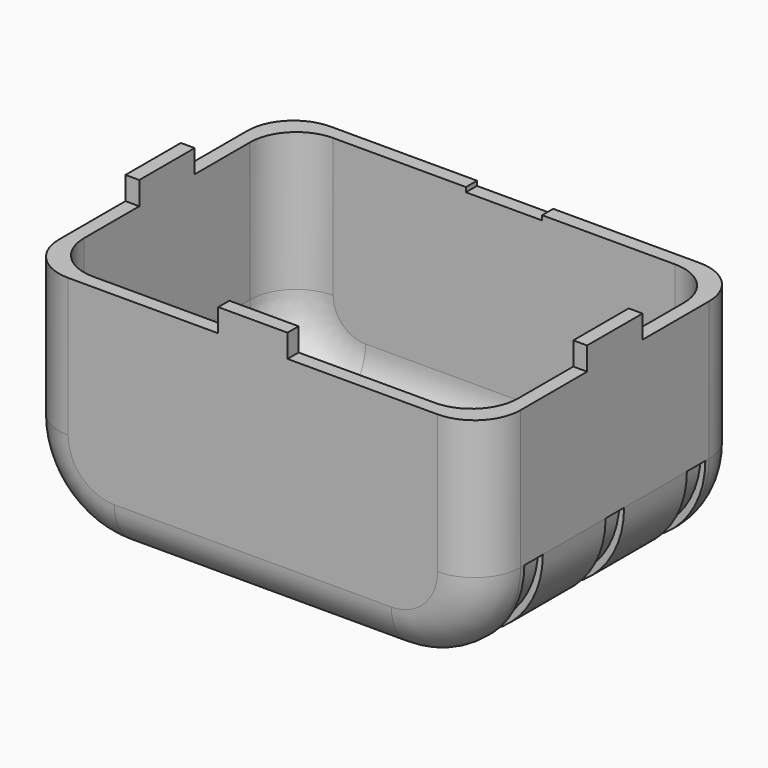
from build123d import *

# Parameters (mm, degrees)
F0_W          = 100
F0_H          = 71
F0_W_2        = 85
F0_H_2        = 56
F1_DEPTH      = 55
F2_R          = 20
F3_T          = -3
F5_DEPTH      = 60
F6_DEPTH      = 55
F7_DEPTH      = 38
F8_DEPTH      = 33
F9_DEPTH      = 16
F10_DEPTH     = 11
F11_W         = 5
F11_H         = 5
F11_W_2       = 7.5
F11_W_3       = 30
F11_W_4       = 5.0000003725
F11_W_5       = 4.9999996275
F11_H_2       = 3
F11_W_6       = 2.5
F12_DEPTH     = 1
F13_R         = 15
F14_DEPTH     = 0.5
F15_W         = 15
F15_H         = 3
F16_DEPTH     = 5
F17_W         = 16.5
F17_H         = 3
F18_DEPTH     = 1
F19_T1_DEPTH  = 60
F19_T3_DEPTH  = 30
F19_T6_ANGLE  = 90
F19_T8_ANGLE  = 90
F19_T10_ANGLE = 90
F19_T12_ANGLE = 90
F19_T13_DEPTH = 60
F19_T15_DEPTH = 55
F19_T18_ANGLE = 90
F19_T20_ANGLE = 90
F19_T22_ANGLE = 90
F19_T24_ANGLE = 90


# Not quite as in the source:
# - a fillet or chamfer that OpenCascade refuses, or shapes differently, is made with other operations: its cross-section is extruded or revolved along the edge and cut away or added
# - ends of sketch curves that miss each other by under 0.0002 mm in the source are joined


with BuildPart() as f1:
    # F0 (on Top) → F1 (new body)
    with BuildSketch(Plane.XY):
        Rectangle(F0_W, F0_H)
        Rectangle(F0_W_2, F0_H_2, mode=Mode.SUBTRACT)
        Rectangle(F0_W_2, F0_H_2)
    extrude(amount=F1_DEPTH)

    # F2
    f2_edges = [f1.edges().sort_by_distance(p)[0] for p in [
        (-50, 0, 0),
        (50, 0, 0),
    ]]
    fillet(f2_edges, radius=F2_R)

    # F3
    f3_openings = [f1.faces().sort_by_distance(p)[0] for p in [
        (0, 0, 55),
    ]]
    offset(amount=F3_T, openings=f3_openings)

    # F4 (on face) → F5 (cut)
    with BuildSketch(Plane(origin=(0, 35.5, 0), x_dir=(-1, 0, 0), z_dir=(0, 1, 0))):
        with BuildLine():
            Line((-49, 21), (-50, 20))
            ThreePointArc((-50, 20), (-44.1421356237, 5.8578643763), (-30, 0))
            Line((-30, 0), (-29, 1))
            ThreePointArc((-29, 1), (-43.1421356237, 6.8578643763), (-49, 21))
        make_face()
        with BuildLine():
            ThreePointArc((30, 0), (44.1421356237, 5.8578643763), (50, 20))
            Line((50, 20), (49, 21))
            ThreePointArc((49, 21), (43.1421356237, 6.8578643763), (29, 1))
            Line((29, 1), (30, 0))
        make_face()
    extrude(amount=-F5_DEPTH, mode=Mode.SUBTRACT)

    # F4 (on face) → F6 (join)
    with BuildSketch(Plane(origin=(0, 35.5, 0), x_dir=(-1, 0, 0), z_dir=(0, 1, 0))):
        with BuildLine():
            Line((-49, 21), (-50, 20))
            ThreePointArc((-50, 20), (-44.1421356237, 5.8578643763), (-30, 0))
            Line((-30, 0), (-29, 1))
            ThreePointArc((-29, 1), (-43.1421356237, 6.8578643763), (-49, 21))
        make_face()
        with BuildLine():
            ThreePointArc((30, 0), (44.1421356237, 5.8578643763), (50, 20))
            Line((50, 20), (49, 21))
            ThreePointArc((49, 21), (43.1421356237, 6.8578643763), (29, 1))
            Line((29, 1), (30, 0))
        make_face()
    extrude(amount=-F6_DEPTH)

    # F4 (on face) → F7 (cut)
    with BuildSketch(Plane(origin=(0, 35.5, 0), x_dir=(-1, 0, 0), z_dir=(0, 1, 0))):
        with BuildLine():
            Line((-49, 21), (-50, 20))
            ThreePointArc((-50, 20), (-44.1421356237, 5.8578643763), (-30, 0))
            Line((-30, 0), (-29, 1))
            ThreePointArc((-29, 1), (-43.1421356237, 6.8578643763), (-49, 21))
        make_face()
        with BuildLine():
            ThreePointArc((30, 0), (44.1421356237, 5.8578643763), (50, 20))
            Line((50, 20), (49, 21))
            ThreePointArc((49, 21), (43.1421356237, 6.8578643763), (29, 1))
            Line((29, 1), (30, 0))
        make_face()
    extrude(amount=-F7_DEPTH, mode=Mode.SUBTRACT)

    # F4 (on face) → F8 (join)
    with BuildSketch(Plane(origin=(0, 35.5, 0), x_dir=(-1, 0, 0), z_dir=(0, 1, 0))):
        with BuildLine():
            Line((-49, 21), (-50, 20))
            ThreePointArc((-50, 20), (-44.1421356237, 5.8578643763), (-30, 0))
            Line((-30, 0), (-29, 1))
            ThreePointArc((-29, 1), (-43.1421356237, 6.8578643763), (-49, 21))
        make_face()
        with BuildLine():
            ThreePointArc((30, 0), (44.1421356237, 5.8578643763), (50, 20))
            Line((50, 20), (49, 21))
            ThreePointArc((49, 21), (43.1421356237, 6.8578643763), (29, 1))
            Line((29, 1), (30, 0))
        make_face()
    extrude(amount=-F8_DEPTH)

    # F4 (on face) → F9 (cut)
    with BuildSketch(Plane(origin=(0, 35.5, 0), x_dir=(-1, 0, 0), z_dir=(0, 1, 0))):
        with BuildLine():
            Line((-49, 21), (-50, 20))
            ThreePointArc((-50, 20), (-44.1421356237, 5.8578643763), (-30, 0))
            Line((-30, 0), (-29, 1))
            ThreePointArc((-29, 1), (-43.1421356237, 6.8578643763), (-49, 21))
        make_face()
        with BuildLine():
            ThreePointArc((30, 0), (44.1421356237, 5.8578643763), (50, 20))
            Line((50, 20), (49, 21))
            ThreePointArc((49, 21), (43.1421356237, 6.8578643763), (29, 1))
            Line((29, 1), (30, 0))
        make_face()
    extrude(amount=-F9_DEPTH, mode=Mode.SUBTRACT)

    # F4 (on face) → F10 (join)
    with BuildSketch(Plane(origin=(0, 35.5, 0), x_dir=(-1, 0, 0), z_dir=(0, 1, 0))):
        with BuildLine():
            Line((-49, 21), (-50, 20))
            ThreePointArc((-50, 20), (-44.1421356237, 5.8578643763), (-30, 0))
            Line((-30, 0), (-29, 1))
            ThreePointArc((-29, 1), (-43.1421356237, 6.8578643763), (-49, 21))
        make_face()
        with BuildLine():
            ThreePointArc((30, 0), (44.1421356237, 5.8578643763), (50, 20))
            Line((50, 20), (49, 21))
            ThreePointArc((49, 21), (43.1421356237, 6.8578643763), (29, 1))
            Line((29, 1), (30, 0))
        make_face()
    extrude(amount=-F10_DEPTH)

    # F11 (on face) → F12 (cut)
    with BuildSketch(Plane(origin=(0, 0, 0), x_dir=(1, 0, 0), z_dir=(0, 0, -1))):
        with Locations((-27.5, 22)):
            Rectangle(F11_W, F11_H)
        with Locations((27.5, 22)):
            Rectangle(F11_W, F11_H)
        with Locations((26.25, 0)):
            Rectangle(F11_W_2, F11_H)
        with Locations((0, 22)):
            Rectangle(F11_W_3, F11_H)
        with Locations((-26.25, 0)):
            Rectangle(F11_W_2, F11_H)
        with Locations((-27.4999998137, -22)):
            Rectangle(F11_W_4, F11_H)
        with Locations((3.725e-07, -21.9999997616)):
            Rectangle(F11_W_3, F11_H)
        with Locations((27.5000001863, -22)):
            Rectangle(F11_W_5, F11_H)
        with Locations((-20, -22)):
            Rectangle(F11_W, F11_H)
        with Locations((-20, -26)):
            Rectangle(F11_W, F11_H_2)
        Polygon((-20, -2.5), (-22.5, -2.5), (-22.5, -19.5), (-17.5, -19.5), (-17.5, -2.5), align=None)
        with Locations((-18.75, 0)):
            Rectangle(F11_W_6, F11_H)
        with Locations((-21.25, 0)):
            Rectangle(F11_W_6, F11_H)
        Polygon((-22.5, 19.5), (-22.5, 2.5), (-20, 2.5), (-17.5, 2.5), (-17.5, 19.5), align=None)
        with Locations((-20, 22)):
            Rectangle(F11_W, F11_H)
        with Locations((-20, 26)):
            Rectangle(F11_W, F11_H_2)
        with Locations((20, 26)):
            Rectangle(F11_W, F11_H_2)
        with Locations((20, 22)):
            Rectangle(F11_W, F11_H)
        Polygon((20, 2.5), (22.5, 2.5), (22.5, 19.5), (17.5, 19.5), (17.5, 2.5), align=None)
        with Locations((21.25, 0)):
            Rectangle(F11_W_6, F11_H)
        with Locations((18.75, 0)):
            Rectangle(F11_W_6, F11_H)
        Polygon((22.5, -19.5), (22.5, -2.5), (20, -2.5), (17.5, -2.5), (17.5, -19.5), align=None)
        with Locations((20, -22)):
            Rectangle(F11_W, F11_H)
        with Locations((20, -26)):
            Rectangle(F11_W, F11_H_2)
    extrude(amount=-F12_DEPTH, mode=Mode.SUBTRACT)

    # F13 (on face) → F14 (cut)
    with BuildSketch(Plane(origin=(0, 0, 0), x_dir=(1, 0, 0), z_dir=(0, 0, -1))):
        Circle(F13_R)
        with BuildLine():
            Line((-6.7133739053, -2.9743209144), (-6.7133739053, -6.2802434318))
            add(Edge.make_bspline(
                [(-6.7133739053, -6.2802434318), (-6.7133739053, -7.4166542972), (-6.0614516847, -7.929642274)],
                knots=[0, 0, 0, 1, 1, 1], degree=2))
            add(Edge.make_bspline(
                [(-6.0614516847, -7.929642274), (-5.4095294642, -8.4426302509), (-4.1519964376, -8.4640047499)],
                knots=[0, 0, 0, 1, 1, 1], degree=2))
            Line((-4.1519964376, -8.4640047499), (-4.1519964376, -10.0243431795))
            add(Edge.make_bspline(
                [(-4.1519964376, -10.0243431795), (-6.2680718421, -9.9994062639), (-7.4258572065, -9.0535846816)],
                knots=[0, 0, 0, 1, 1, 1], degree=2))
            add(Edge.make_bspline(
                [(-7.4258572065, -9.0535846816), (-8.5836425709, -8.1077630993), (-8.5836425709, -6.39424076)],
                knots=[0, 0, 0, 1, 1, 1], degree=2))
            Line((-8.5836425709, -6.39424076), (-8.5836425709, -3.0206323289))
            add(Edge.make_bspline(
                [(-8.5836425709, -3.0206323289), (-8.5836425709, -1.8628469645), (-9.2836574143, -1.3676710702)],
                knots=[0, 0, 0, 1, 1, 1], degree=2))
            add(Edge.make_bspline(
                [(-9.2836574143, -1.3676710702), (-9.9836722577, -0.8724951759), (-11.3195784474, -0.8724951759)],
                knots=[0, 0, 0, 1, 1, 1], degree=2))
            Line((-11.3195784474, -0.8724951759), (-11.3195784474, 0.6985305032))
            add(Edge.make_bspline(
                [(-11.3195784474, 0.6985305032), (-9.873237346, 0.7199050022), (-9.2284399584, 1.2328929791)],
                knots=[0, 0, 0, 1, 1, 1], degree=2))
            add(Edge.make_bspline(
                [(-9.2284399584, 1.2328929791), (-8.5836425709, 1.7458809559), (-8.5836425709, 2.8146059077)],
                knots=[0, 0, 0, 1, 1, 1], degree=2))
            Line((-8.5836425709, 2.8146059077), (-8.5836425709, 6.2202760873))
            add(Edge.make_bspline(
                [(-8.5836425709, 6.2202760873), (-8.5836425709, 7.9444856761), (-7.3813270001, 8.9027757162)],
                knots=[0, 0, 0, 1, 1, 1], degree=2))
            add(Edge.make_bspline(
                [(-7.3813270001, 8.9027757162), (-6.1790114294, 9.8610657563), (-4.1519964376, 9.8610657563)],
                knots=[0, 0, 0, 1, 1, 1], degree=2))
            Line((-4.1519964376, 9.8610657563), (-4.1519964376, 8.3114145762))
            add(Edge.make_bspline(
                [(-4.1519964376, 8.3114145762), (-6.7133739053, 8.2472910791), (-6.7133739053, 6.0991539261)],
                knots=[0, 0, 0, 1, 1, 1], degree=2))
            Line((-6.7133739053, 6.0991539261), (-6.7133739053, 2.8146059077))
            add(Edge.make_bspline(
                [(-6.7133739053, 2.8146059077), (-6.7133739053, 0.4206620157), (-9.1928157934, -0.013952798)],
                knots=[0, 0, 0, 1, 1, 1], degree=2))
            Line((-9.1928157934, -0.013952798), (-9.1928157934, -0.1493246252))
            add(Edge.make_bspline(
                [(-9.1928157934, -0.1493246252), (-6.7133739053, -0.5803770224), (-6.7133739053, -2.9743209144)],
                knots=[0, 0, 0, 1, 1, 1], degree=2))
        make_face(mode=Mode.SUBTRACT)
        with BuildLine():
            Line((8.373459997, -0.1493246252), (8.373459997, -0.013952798))
            add(Edge.make_bspline(
                [(8.373459997, -0.013952798), (5.8904556924, 0.4206620157), (5.8904556924, 2.8146059077)],
                knots=[0, 0, 0, 1, 1, 1], degree=2))
            Line((5.8904556924, 2.8146059077), (5.8904556924, 6.0991539261))
            add(Edge.make_bspline(
                [(5.8904556924, 6.0991539261), (5.8904556924, 8.2472910791), (3.3647023898, 8.3114145762)],
                knots=[0, 0, 0, 1, 1, 1], degree=2))
            Line((3.3647023898, 8.3114145762), (3.3647023898, 9.8610657563))
            add(Edge.make_bspline(
                [(3.3647023898, 9.8610657563), (5.4130918807, 9.8610657563), (6.5869081193, 8.8920884667)],
                knots=[0, 0, 0, 1, 1, 1], degree=2))
            add(Edge.make_bspline(
                [(6.5869081193, 8.8920884667), (7.760724358, 7.9231111771), (7.760724358, 6.2202760873)],
                knots=[0, 0, 0, 1, 1, 1], degree=2))
            Line((7.760724358, 6.2202760873), (7.760724358, 2.8146059077))
            add(Edge.make_bspline(
                [(7.760724358, 2.8146059077), (7.760724358, 1.7351937064), (8.4179902034, 1.2275493543)],
                knots=[0, 0, 0, 1, 1, 1], degree=2))
            add(Edge.make_bspline(
                [(8.4179902034, 1.2275493543), (9.0752560487, 0.7199050022), (10.5215971501, 0.6985305032)],
                knots=[0, 0, 0, 1, 1, 1], degree=2))
            Line((10.5215971501, 0.6985305032), (10.5215971501, -0.8724951759))
            add(Edge.make_bspline(
                [(10.5215971501, -0.8724951759), (9.1643164613, -0.8724951759), (8.4625204097, -1.3676710702)],
                knots=[0, 0, 0, 1, 1, 1], degree=2))
            add(Edge.make_bspline(
                [(8.4625204097, -1.3676710702), (7.760724358, -1.8628469645), (7.760724358, -3.0206323289)],
                knots=[0, 0, 0, 1, 1, 1], degree=2))
            Line((7.760724358, -3.0206323289), (7.760724358, -6.39424076))
            add(Edge.make_bspline(
                [(7.760724358, -6.39424076), (7.760724358, -8.0970758498), (6.6207510761, -9.0482410569)],
                knots=[0, 0, 0, 1, 1, 1], degree=2))
            add(Edge.make_bspline(
                [(6.6207510761, -9.0482410569), (5.4807777943, -9.9994062639), (3.3647023898, -10.0243431795)],
                knots=[0, 0, 0, 1, 1, 1], degree=2))
            Line((3.3647023898, -10.0243431795), (3.3647023898, -8.4640047499))
            add(Edge.make_bspline(
                [(3.3647023898, -8.4640047499), (4.6008609173, -8.4426302509), (5.2456583049, -7.929642274)],
                knots=[0, 0, 0, 1, 1, 1], degree=2))
            add(Edge.make_bspline(
                [(5.2456583049, -7.929642274), (5.8904556924, -7.4166542972), (5.8904556924, -6.2802434318)],
                knots=[0, 0, 0, 1, 1, 1], degree=2))
            Line((5.8904556924, -6.2802434318), (5.8904556924, -2.9743209144))
            add(Edge.make_bspline(
                [(5.8904556924, -2.9743209144), (5.8904556924, -1.7061006383), (6.5031913315, -1.0381475434)],
                knots=[0, 0, 0, 1, 1, 1], degree=2))
            add(Edge.make_bspline(
                [(6.5031913315, -1.0381475434), (7.1159269705, -0.3701944486), (8.373459997, -0.1493246252)],
                knots=[0, 0, 0, 1, 1, 1], degree=2))
        make_face(mode=Mode.SUBTRACT)
    extrude(amount=-F14_DEPTH, mode=Mode.SUBTRACT)

    # F15 (on face) → F16 (cut)
    with BuildSketch(Plane.XY.offset(55)):
        Polygon((50, 35.5), (7.5, 35.5), (7.5, 32.5), (47, 32.5), (47, 7.5), (50, 7.5), align=None)
        Polygon((-7.5, 32.5), (-7.5, 35.5), (-50, 35.5), (-50, 7.5), (-47, 7.5), (-47, 32.5), align=None)
        Polygon((-47, -7.5), (-50, -7.5), (-50, -35.5), (-7.5, -35.5), (-7.5, -32.5), (-47, -32.5), align=None)
        Polygon((50, -35.5), (50, -7.5), (47, -7.5), (47, -32.5), (7.5, -32.5), (7.5, -35.5), align=None)
        with Locations((0, 34)):
            Rectangle(F15_W, F15_H)
    extrude(amount=-F16_DEPTH, mode=Mode.SUBTRACT)

    # F17 (on face) → F18 (cut)
    with BuildSketch(Plane.XY.offset(50)):
        with Locations((0, 34)):
            Rectangle(F17_W, F17_H)
    extrude(amount=-F18_DEPTH, mode=Mode.SUBTRACT)

    # F19: fillet of radius 10 on 4 edges, made by hand

    # F19_s2 → F19_t1 (join)
    with BuildSketch(Plane.YZ.offset(-30)):
        with BuildLine():
            ThreePointArc((-32.5, 13), (-29.5710678119, 5.9289321881), (-22.5, 3))
            Line((-22.5, 3), (-32.5, 3))
            Line((-32.5, 3), (-32.5, 13))
        make_face()
        with BuildLine():
            ThreePointArc((32.5, 13), (29.5710678119, 5.9289321881), (22.5, 3))
            Line((22.5, 3), (32.5, 3))
            Line((32.5, 3), (32.5, 13))
        make_face()
    extrude(amount=F19_T1_DEPTH)

    # F19_s4 → F19_t3 (join)
    with BuildSketch(Plane.XY.offset(20)):
        with BuildLine():
            ThreePointArc((-37, 32.5), (-44.0710678119, 29.5710678119), (-47, 22.5))
            Line((-47, 22.5), (-47, 32.5))
            Line((-47, 32.5), (-37, 32.5))
        make_face()
        with BuildLine():
            ThreePointArc((47, 22.5), (44.0710678119, 29.5710678119), (37, 32.5))
            Line((37, 32.5), (47, 32.5))
            Line((47, 32.5), (47, 22.5))
        make_face()
        with BuildLine():
            ThreePointArc((47, -22.5), (44.0710678119, -29.5710678119), (37, -32.5))
            Line((37, -32.5), (47, -32.5))
            Line((47, -32.5), (47, -22.5))
        make_face()
        with BuildLine():
            ThreePointArc((-37, -32.5), (-44.0710678119, -29.5710678119), (-47, -22.5))
            Line((-47, -22.5), (-47, -32.5))
            Line((-47, -32.5), (-37, -32.5))
        make_face()
    extrude(amount=F19_T3_DEPTH)

    # F19_s5 → F19_t6 (revolve)
    with BuildSketch(Plane.XY.offset(20)):
        with BuildLine():
            ThreePointArc((37, 32.5), (44.0710678119, 29.5710678119), (47, 22.5))
            Line((47, 22.5), (47, 32.5))
            Line((47, 32.5), (37, 32.5))
        make_face()
    revolve(axis=Axis((30, 32.5, 20), (0, 1, 0)), revolution_arc=F19_T6_ANGLE)

    # F19_s7 → F19_t8 (revolve)
    with BuildSketch(Plane.XY.offset(20)):
        with BuildLine():
            ThreePointArc((-37, 32.5), (-44.0710678119, 29.5710678119), (-47, 22.5))
            Line((-47, 22.5), (-47, 32.5))
            Line((-47, 32.5), (-37, 32.5))
        make_face()
    revolve(axis=Axis((-30, 32.5, 20), (0, -1, 0)), revolution_arc=F19_T8_ANGLE)

    # F19_s9 → F19_t10 (revolve)
    with BuildSketch(Plane.XY.offset(20)):
        with BuildLine():
            ThreePointArc((-37, -32.5), (-44.0710678119, -29.5710678119), (-47, -22.5))
            Line((-47, -22.5), (-47, -32.5))
            Line((-47, -32.5), (-37, -32.5))
        make_face()
    revolve(axis=Axis((-30, -32.5, 20), (0, -1, 0)), revolution_arc=F19_T10_ANGLE)

    # F19_s11 → F19_t12 (revolve)
    with BuildSketch(Plane.XY.offset(20)):
        with BuildLine():
            ThreePointArc((37, -32.5), (44.0710678119, -29.5710678119), (47, -22.5))
            Line((47, -22.5), (47, -32.5))
            Line((47, -32.5), (37, -32.5))
        make_face()
    revolve(axis=Axis((30, -32.5, 20), (0, 1, 0)), revolution_arc=F19_T12_ANGLE)

    # F19_s14 → F19_t13 (cut)
    with BuildSketch(Plane.YZ.offset(-30)):
        with BuildLine():
            ThreePointArc((35.5, 10), (32.5710678119, 2.9289321881), (25.5, 0))
            Line((25.5, 0), (35.5, 0))
            Line((35.5, 0), (35.5, 10))
        make_face()
        with BuildLine():
            ThreePointArc((-35.5, 10), (-32.5710678119, 2.9289321881), (-25.5, 0))
            Line((-25.5, 0), (-35.5, 0))
            Line((-35.5, 0), (-35.5, 10))
        make_face()
    extrude(amount=F19_T13_DEPTH, mode=Mode.SUBTRACT)

    # F19_s16 → F19_t15 (cut)
    with BuildSketch(Plane.XY.offset(20)):
        with BuildLine():
            ThreePointArc((50, -25.5), (47.0710678119, -32.5710678119), (40, -35.5))
            Line((40, -35.5), (50, -35.5))
            Line((50, -35.5), (50, -25.5))
        make_face()
        with BuildLine():
            ThreePointArc((-40, -35.5), (-47.0710678119, -32.5710678119), (-50, -25.5))
            Line((-50, -25.5), (-50, -35.5))
            Line((-50, -35.5), (-40, -35.5))
        make_face()
        with BuildLine():
            ThreePointArc((-40, 35.5), (-47.0710678119, 32.5710678119), (-50, 25.5))
            Line((-50, 25.5), (-50, 35.5))
            Line((-50, 35.5), (-40, 35.5))
        make_face()
        with BuildLine():
            ThreePointArc((50, 25.5), (47.0710678119, 32.5710678119), (40, 35.5))
            Line((40, 35.5), (50, 35.5))
            Line((50, 35.5), (50, 25.5))
        make_face()
    extrude(amount=F19_T15_DEPTH, mode=Mode.SUBTRACT)

    # F19_s17 → F19_t18 (revolve, cut)
    with BuildSketch(Plane.XY.offset(20)):
        with BuildLine():
            ThreePointArc((-40, -35.5), (-47.0710678119, -32.5710678119), (-50, -25.5))
            Line((-50, -25.5), (-50, -35.5))
            Line((-50, -35.5), (-40, -35.5))
        make_face()
    revolve(axis=Axis((-30, -35.5, 20), (0, -1, 0)), revolution_arc=F19_T18_ANGLE, mode=Mode.SUBTRACT)

    # F19_s19 → F19_t20 (revolve, cut)
    with BuildSketch(Plane.XY.offset(20)):
        with BuildLine():
            ThreePointArc((50, -25.5), (47.0710678119, -32.5710678119), (40, -35.5))
            Line((40, -35.5), (50, -35.5))
            Line((50, -35.5), (50, -25.5))
        make_face()
    revolve(axis=Axis((30, -35.5, 20), (0, 1, 0)), revolution_arc=F19_T20_ANGLE, mode=Mode.SUBTRACT)

    # F19_s21 → F19_t22 (revolve, cut)
    with BuildSketch(Plane.XY.offset(20)):
        with BuildLine():
            ThreePointArc((50, 25.5), (47.0710678119, 32.5710678119), (40, 35.5))
            Line((40, 35.5), (50, 35.5))
            Line((50, 35.5), (50, 25.5))
        make_face()
    revolve(axis=Axis((30, 35.5, 20), (0, 1, 0)), revolution_arc=F19_T22_ANGLE, mode=Mode.SUBTRACT)

    # F19_s23 → F19_t24 (revolve, cut)
    with BuildSketch(Plane.YZ.offset(-30)):
        with BuildLine():
            ThreePointArc((35.5, 10), (32.5710678119, 2.9289321881), (25.5, 0))
            Line((25.5, 0), (35.5, 0))
            Line((35.5, 0), (35.5, 10))
        make_face()
    revolve(axis=Axis((-30, 35.5, 20), (0, 1, 0)), revolution_arc=F19_T24_ANGLE, mode=Mode.SUBTRACT)


solid = f1.part
